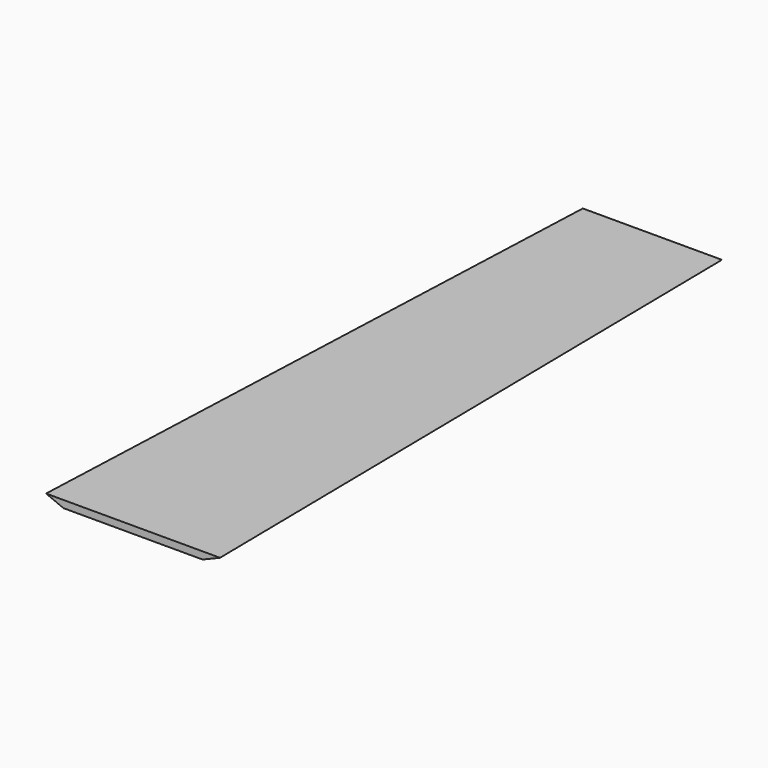
from build123d import *

# Parameters (mm, degrees)
F1_DEPTH = 177.8
F3_DEPTH = 25.4


# Not quite as in the source:
# - a feature names something its author has since deleted; it is built from what else it names


with BuildPart() as f1:
    # F0 (on Front) → F1 (new body)
    with BuildSketch(Plane.XZ):
        Polygon((0, 1.9812), (0, 0), (19.05, 0), (23.8252, 1.9812), align=None)
        Polygon((-19.05, 0), (0, 0), (0, 1.9812), (-23.8252, 1.9812), align=None)
    extrude(amount=F1_DEPTH)

    # F2 (on Right) → F3 (cut, symmetric)
    with BuildSketch(Plane.YZ):
        Polygon((-177.7999848127, 1.9810541999), (0, 0), (0, 5.3311795928), (-177.7999848127, 1.9878952298), align=None)
    extrude(amount=F3_DEPTH, both=True, mode=Mode.SUBTRACT)


solid = f1.part
